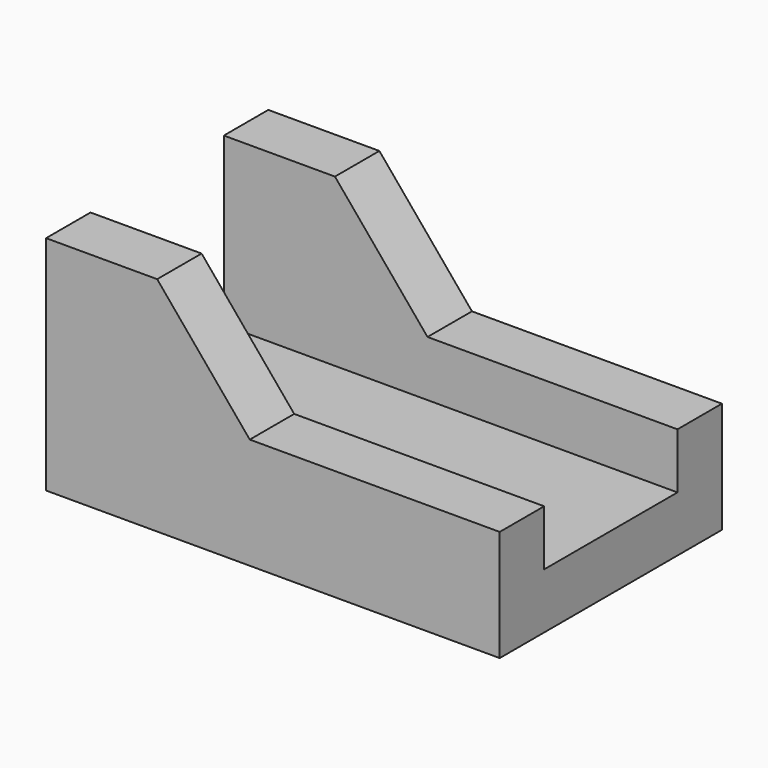
from build123d import *

# Parameters (mm, degrees)
F0_W     = 77.7875
F0_H     = 47.625
F1_DEPTH = 9.525
F3_DEPTH = 9.525


# Not quite as in the source:
# - a pattern or mirror of a feature is missing from the dataset's text; its kind, count and spacing are read off the source's solid


with BuildPart() as f1:
    # F0 (on Top) → F1 (new body)
    with BuildSketch(Plane.XY):
        Rectangle(F0_W, F0_H)
    extrude(amount=F1_DEPTH)

    # F2 (on face) → F3 (join)
    with BuildSketch(Plane.XZ.offset(23.8125)):
        Polygon((-38.89375, 38.1), (-38.89375, 0), (38.89375, 0), (38.89375, 9.525), (38.89375, 19.05), (-3.96875, 19.05), (-19.84375, 38.1), align=None)
    f3 = extrude(amount=-F3_DEPTH)

    # F3_copies: F3 across plane
    add(f3.mirror(Plane.ZX))


solid = f1.part
